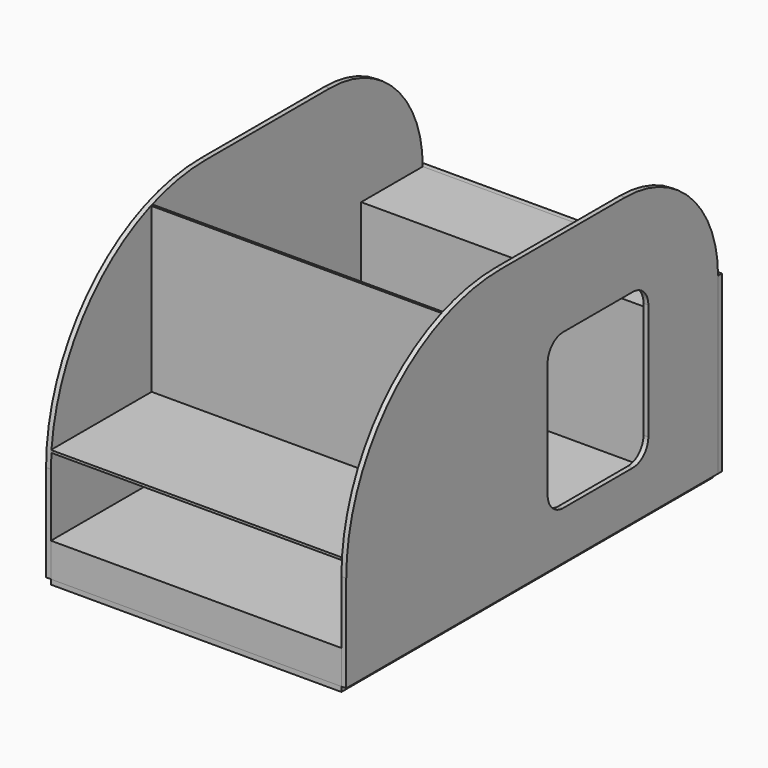
from build123d import *

# Parameters (mm, degrees)
F0_W      = 2438.4
F0_H      = 1524
F1_DEPTH  = 25.4
F3_DEPTH  = 25.401
F4_W      = 1524
F4_H      = 2438.4
F5_DEPTH  = 25.4
F8_W      = 1574.782686615
F8_H      = 914.4
F9_DEPTH  = 25.4
F11_DEPTH = 1574.8
F12_W     = 1524
F12_H     = 2032
F13_DEPTH = 177.8
F15_W     = 1524
F15_H     = 660.4
F16_DEPTH = 12.7
F17_W     = 1524
F17_H     = 870.994234848
F18_DEPTH = 12.7
F19_W     = 1524
F19_H     = 403.904914856
F20_DEPTH = 914.4


with BuildPart() as f1:
    # F0 (on Right) → F1 (new body)
    with BuildSketch(Plane.YZ):
        with Locations((-1219.2, 762)):
            Rectangle(F0_W, F0_H)
    extrude(amount=F1_DEPTH)

    # F2 (on face) → F3 (cut, through all)
    with BuildSketch(Plane.YZ.offset(25.4)):
        with BuildLine():
            ThreePointArc((-2438.4, 508), (-2140.8204896855, 1226.4204896855), (-1422.4, 1524))
            Line((-1422.4, 1524), (-2438.4, 1524))
            Line((-2438.4, 1524), (-2438.4, 508))
        make_face()
        with BuildLine():
            ThreePointArc((-609.6, 1524), (-178.5477061887, 1345.4522938113), (0, 914.4))
            Line((0, 914.4), (0, 1524))
            Line((0, 1524), (-609.6, 1524))
        make_face()
    extrude(amount=-F3_DEPTH, mode=Mode.SUBTRACT)


with BuildPart() as f5:
    # F4 (on Top) → F5 (new body)
    with BuildSketch(Plane.XY):
        with Locations((-762, -1219.2)):
            Rectangle(F4_W, F4_H)
    extrude(amount=-F5_DEPTH)


with BuildPart() as f7_1:
    # F7: instance of F1
    add(f1.part.mirror(Plane.YZ.offset(-762)))


with BuildPart() as f9:
    # F8 (on face) → F9 (new body)
    with BuildSketch(Plane(origin=(0, 0, 0), x_dir=(-1, 0, 0), z_dir=(0, 1, 0))):
        with Locations((761.9913433075, 457.2)):
            Rectangle(F8_W, F8_H)
    extrude(amount=F9_DEPTH)


with BuildPart() as f1_1:
    add(f1.part)

    # F10 (on face) → F11 (cut)
    with BuildSketch(Plane.YZ.offset(25.4)):
        with BuildLine():
            Line((-558.8, 1066.8), (-1016, 1066.8))
            ThreePointArc((-1016, 1066.8), (-1087.8420489686, 1037.0420489686), (-1117.6, 965.2))
            Line((-1117.6, 965.2), (-1117.6, 355.6))
            ThreePointArc((-1117.6, 355.6), (-1087.8420489686, 283.7579510314), (-1016, 254))
            Line((-1016, 254), (-558.8, 254))
            ThreePointArc((-558.8, 254), (-486.9579510314, 283.7579510314), (-457.2, 355.6))
            Line((-457.2, 355.6), (-457.2, 965.2))
            ThreePointArc((-457.2, 965.2), (-486.9579510314, 1037.0420489686), (-558.8, 1066.8))
        make_face()
    extrude(amount=-F11_DEPTH, mode=Mode.SUBTRACT)


with BuildPart() as f13:
    # F12 (on face) → F13 (new body)
    with BuildSketch(Plane.XY):
        with Locations((-762, -1422.4)):
            Rectangle(F12_W, F12_H)
    extrude(amount=F13_DEPTH)


with BuildPart() as f16:
    # F15 (on offset) → F16 (new body)
    with BuildSketch(Plane.XY.offset(584.2)):
        with Locations((-762, -2108.2)):
            Rectangle(F15_W, F15_H)
    extrude(amount=F16_DEPTH)


with BuildPart() as f18:
    # F17 (on face) → F18 (new body)
    with BuildSketch(Plane(origin=(0, -1778, 0), x_dir=(-1, 0, 0), z_dir=(0, 1, 0))):
        with Locations((762, 1019.697117424)):
            Rectangle(F17_W, F17_H)
    extrude(amount=F18_DEPTH)


with BuildPart() as f20:
    # F19 (on face) → F20 (new body)
    with BuildSketch(Plane.XY):
        with Locations((-762, -201.952457428)):
            Rectangle(F19_W, F19_H)
    extrude(amount=F20_DEPTH)


solid = Compound([f5.part, f7_1.part, f9.part, f1_1.part, f13.part, f16.part, f18.part, f20.part])
